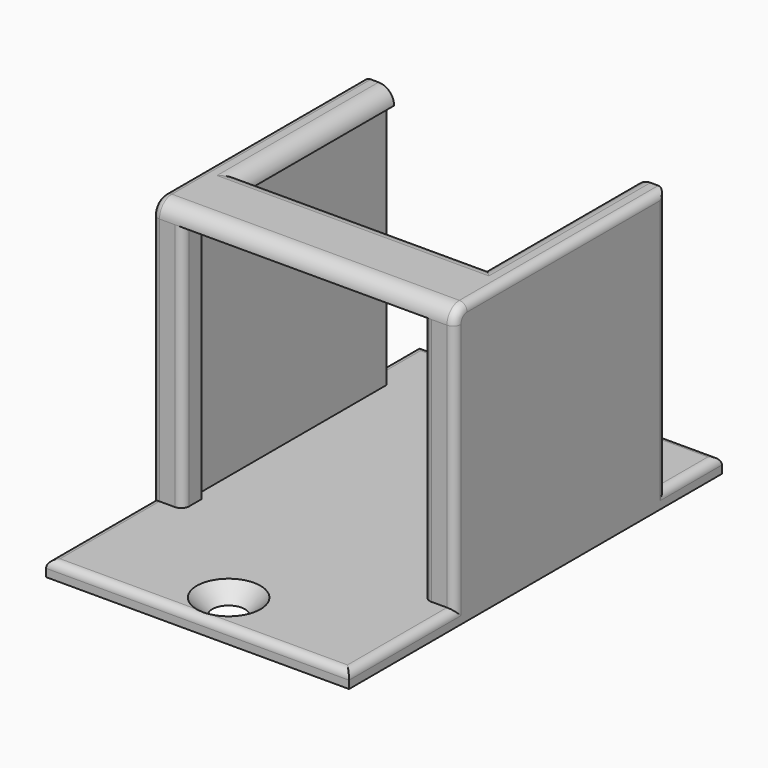
from build123d import *

# Parameters (mm, degrees)
F0_W          = 3
F0_H          = 9
F0_H_2        = 7
F0_H_3        = 3
F0_R          = 2.1
F0_W_2        = 1
F1_DEPTH      = 2
F2_DEPTH      = 34
F3_W          = 4
F3_H          = 2
F4_DEPTH      = 34
F5_SIZE       = 1.99999
F7_W          = 1
F7_H          = 1
F8_DEPTH      = 1
F3_W_2        = 31
F9_DEPTH      = 10
F10_R         = 1.99999
F11_T1_DEPTH  = 32
F11_T3_DEPTH  = 34.50001
F11_T5_DEPTH  = 32.00001
F11_T7_DEPTH  = 19.5
F11_T9_DEPTH  = 11.5
F11_T11_DEPTH = 44
F11_T13_DEPTH = 36.5
F11_T16_ANGLE = 90
F11_T18_ANGLE = 90
F11_T23_DEPTH = 34.50001
F11_T27_DEPTH = 22
F11_T34_DEPTH = 14
F11_T38_DEPTH = 39
F11_T45_DEPTH = 22
F11_T49_DEPTH = 34.50001


# Not quite as in the source:
# - a fillet or chamfer that OpenCascade refuses, or shapes differently, is made with other operations: its cross-section is extruded or revolved along the edge and cut away or added
# - a fillet or chamfer is up to 0.001 mm smaller than in the source, because OpenCascade refuses the exact size
# - a feature of the source that left no trace in its solid (it failed there, or was rolled back) is left out
# - a feature names something its author has since deleted; it is built from what else it names


with BuildPart() as f1:
    # F0 (on Top) → F1 (new body)
    with BuildSketch(Plane.XY):
        with Locations((18, 20.5)):
            Rectangle(F0_W, F0_H)
        with Locations((-18, 20.5)):
            Rectangle(F0_W, F0_H)
        with Locations((18, -21.5)):
            Rectangle(F0_W, F0_H_2)
        with Locations((-18, -21.5)):
            Rectangle(F0_W, F0_H_2)
        with Locations((18, -16.5)):
            Rectangle(F0_W, F0_H_3)
        with Locations((-18, -16.5)):
            Rectangle(F0_W, F0_H_3)
        Polygon((19.5, -35), (19.5, -25), (16.5, -25), (-16.5, -25), (-19.5, -25), (-19.5, -35), align=None)
        with Locations((0, -30)):
            Circle(F0_R, mode=Mode.SUBTRACT)
        Polygon((19.5, -15), (19.5, 16), (16.5, 16), (16.5, 15), (16.5, -15), align=None)
        Polygon((-16.5, 15), (-16.5, 16), (-19.5, 16), (-19.5, 15), (-19.5, -15), (-16.5, -15), align=None)
        Polygon((16.5, 16), (16.5, 25), (-16.5, 25), (-16.5, 16), (-16.5, 15), (16.5, 15), align=None)
        with Locations((0, 20)):
            Circle(F0_R, mode=Mode.SUBTRACT)
        Polygon((16.5, -15), (16.5, 15), (-16.5, 15), (-16.5, -15), (-15.5, -15), (15.5, -15), align=None)
        with Locations((-16, -16.5)):
            Rectangle(F0_W_2, F0_H_3)
        with Locations((16, -16.5)):
            Rectangle(F0_W_2, F0_H_3)
        Polygon((16.5, -25), (16.5, -18), (15.5, -18), (15.5, -15), (-15.5, -15), (-15.5, -18), (-16.5, -18), (-16.5, -25), align=None)
        with Locations((0, -20)):
            Circle(F0_R, mode=Mode.SUBTRACT)
        with Locations((0, -20)):
            Circle(F0_R)
    extrude(amount=-F1_DEPTH)

    # F0 (on Top) → F2 (join)
    with BuildSketch(Plane.XY):
        Polygon((-16.5, 15), (-16.5, 16), (-19.5, 16), (-19.5, 15), (-19.5, -15), (-16.5, -15), align=None)
        with Locations((-18, -16.5)):
            Rectangle(F0_W, F0_H_3)
        with Locations((18, -16.5)):
            Rectangle(F0_W, F0_H_3)
        with Locations((16, -16.5)):
            Rectangle(F0_W_2, F0_H_3)
        with Locations((-16, -16.5)):
            Rectangle(F0_W_2, F0_H_3)
        Polygon((19.5, -15), (19.5, 16), (16.5, 16), (16.5, 15), (16.5, -15), align=None)
    extrude(amount=F2_DEPTH)

    # F3 (on face) → F4 (join)
    with BuildSketch(Plane.XZ.offset(18)):
        with Locations((-17.5, 33)):
            Rectangle(F3_W, F3_H)
        with Locations((17.5, 33)):
            Rectangle(F3_W, F3_H)
    extrude(amount=-F4_DEPTH)

    # F5 (size 2 in the source; OpenCascade refuses exactly that, so slightly less here)
    f5_edges = [f1.edges().sort_by_distance(p)[0] for p in [
        (-2.1, -30, 0),
        (-2.1, 20, 0),
    ]]
    chamfer(f5_edges, length=F5_SIZE)

    # F7 (on face) → F8 (join)
    with BuildSketch(Plane(origin=(0, 16, 0), x_dir=(-1, 0, 0), z_dir=(0, 1, 0))):
        with Locations((-16, 31.5)):
            Rectangle(F7_W, F7_H)
        Polygon((15.9987417102, 33.0025165796), (15.5, 34), (15.5050715785, 33.0000128605), align=None)
    extrude(amount=-F8_DEPTH)

    # F3 (on face) → F9 (join)
    with BuildSketch(Plane.XZ.offset(18)):
        with Locations((0, 33)):
            Rectangle(F3_W_2, F3_H)
    extrude(amount=-F9_DEPTH)

    # F10 (radius 2 in the source; OpenCascade refuses exactly that, so slightly less here)
    f10_edges = [f1.edges().sort_by_distance(p)[0] for p in [
        (0, -18, 34),
        (-15.5, 4, 34),
        (0, -8, 34),
        (15.5, 4, 34),
    ]]
    fillet(f10_edges, radius=F10_R)

    # F11: fillet of radius 1 on 15 edges, made by hand

    # F11_s2 → F11_t1 (cut)
    with BuildSketch(Plane.XY):
        with BuildLine():
            ThreePointArc((-16.5, -18), (-15.7928932188, -17.7071067812), (-15.5, -17))
            Line((-15.5, -17), (-15.5, -18))
            Line((-15.5, -18), (-16.5, -18))
        make_face()
        with BuildLine():
            ThreePointArc((15.5, -17), (15.7928932188, -17.7071067812), (16.5, -18))
            Line((16.5, -18), (15.5, -18))
            Line((15.5, -18), (15.5, -17))
        make_face()
    extrude(amount=F11_T1_DEPTH, mode=Mode.SUBTRACT)

    # F11_s4 → F11_t3 (cut)
    with BuildSketch(Plane.XZ.offset(-18.5)):
        with BuildLine():
            ThreePointArc((-18.5, 34), (-19.2071067812, 33.7071067812), (-19.5, 33))
            Line((-19.5, 33), (-19.5, 34))
            Line((-19.5, 34), (-18.5, 34))
        make_face()
        with BuildLine():
            ThreePointArc((18.5, 34), (19.2071067812, 33.7071067812), (19.5, 33))
            Line((19.5, 33), (19.5, 34))
            Line((19.5, 34), (18.5, 34))
        make_face()
    extrude(amount=F11_T3_DEPTH, mode=Mode.SUBTRACT)

    # F11_s6 → F11_t5 (cut)
    with BuildSketch(Plane.XY):
        with BuildLine():
            ThreePointArc((-19.5, -17), (-19.2071067812, -17.7071067812), (-18.5, -18))
            Line((-18.5, -18), (-19.5, -18))
            Line((-19.5, -18), (-19.5, -17))
        make_face()
        with BuildLine():
            ThreePointArc((18.5, -18), (19.2071067812, -17.7071067812), (19.5, -17))
            Line((19.5, -17), (19.5, -18))
            Line((19.5, -18), (18.5, -18))
        make_face()
    extrude(amount=F11_T5_DEPTH, mode=Mode.SUBTRACT)

    # F11_s8 → F11_t7 (cut)
    with BuildSketch(Plane.XZ.offset(18)):
        with BuildLine():
            ThreePointArc((-19.5, -1), (-19.2071067812, -0.2928932188), (-18.5, 0))
            Line((-18.5, 0), (-19.5, 0))
            Line((-19.5, 0), (-19.5, -1))
        make_face()
        with BuildLine():
            ThreePointArc((18.5, 0), (19.2071067812, -0.2928932188), (19.5, -1))
            Line((19.5, -1), (19.5, 0))
            Line((19.5, 0), (18.5, 0))
        make_face()
    extrude(amount=F11_T7_DEPTH, mode=Mode.SUBTRACT)

    # F11_s10 → F11_t9 (cut)
    with BuildSketch(Plane.XZ.offset(-27.5)):
        with BuildLine():
            ThreePointArc((-19.5, -1), (-19.2071067812, -0.2928932188), (-18.5, 0))
            Line((-18.5, 0), (-19.5, 0))
            Line((-19.5, 0), (-19.5, -1))
        make_face()
        with BuildLine():
            ThreePointArc((18.5, 0), (19.2071067812, -0.2928932188), (19.5, -1))
            Line((19.5, -1), (19.5, 0))
            Line((19.5, 0), (18.5, 0))
        make_face()
    extrude(amount=F11_T9_DEPTH, mode=Mode.SUBTRACT)

    # F11_s12 → F11_t11 (cut)
    with BuildSketch(Plane.YZ.offset(-22)):
        with BuildLine():
            ThreePointArc((-34, 0), (-34.7071067812, -0.2928932188), (-35, -1))
            Line((-35, -1), (-35, 0))
            Line((-35, 0), (-34, 0))
        make_face()
        with BuildLine():
            ThreePointArc((24, 0), (24.7071067812, -0.2928932188), (25, -1))
            Line((25, -1), (25, 0))
            Line((25, 0), (24, 0))
        make_face()
    extrude(amount=F11_T11_DEPTH, mode=Mode.SUBTRACT)

    # F11_s14 → F11_t13 (cut)
    with BuildSketch(Plane.XY):
        with BuildLine():
            ThreePointArc((19.5, 15), (19.2071067812, 15.7071067812), (18.5, 16))
            Line((18.5, 16), (19.5, 16))
            Line((19.5, 16), (19.5, 15))
        make_face()
    extrude(amount=F11_T13_DEPTH, mode=Mode.SUBTRACT)

    # F11_s15 → F11_t16 (revolve, cut)
    with BuildSketch(Plane.XZ.offset(16.00001)):
        with BuildLine():
            ThreePointArc((-19.5, 33), (-19.2071067812, 33.7071067812), (-18.5, 34))
            Line((-18.5, 34), (-19.5, 34))
            Line((-19.5, 34), (-19.5, 33))
        make_face()
    revolve(axis=Axis((-19.5, -16.00001, 32.00001), (1, 0, 0)), revolution_arc=F11_T16_ANGLE, mode=Mode.SUBTRACT)

    # F11_s17 → F11_t18 (revolve, cut)
    with BuildSketch(Plane.XZ.offset(16.00001)):
        with BuildLine():
            ThreePointArc((18.5, 34), (19.2071067812, 33.7071067812), (19.5, 33))
            Line((19.5, 33), (19.5, 34))
            Line((19.5, 34), (18.5, 34))
        make_face()
    revolve(axis=Axis((19.5, -16.00001, 32.00001), (1, 0, 0)), revolution_arc=F11_T18_ANGLE, mode=Mode.SUBTRACT)


with BuildPart() as f11_tool21:
    # F11_s22 → F11_t23 (new body)
    with BuildSketch(Plane.XY.offset(-2.5)):
        with BuildLine():
            ThreePointArc((-19.5, -17), (-19.2071067812, -17.7071067812), (-18.5, -18))
            Line((-18.5, -18), (-19.5, -18))
            Line((-19.5, -18), (-19.5, -17))
        make_face()
    extrude(amount=F11_T23_DEPTH)

    split(bisect_by=Plane.XY, keep=Keep.BOTTOM)


with BuildPart() as f11_tool25:
    # F11_s26 → F11_t27 (new body)
    with BuildSketch(Plane.XZ.offset(15.5)):
        with BuildLine():
            ThreePointArc((-19.5, -1), (-19.2071067812, -0.2928932188), (-18.5, 0))
            Line((-18.5, 0), (-19.5, 0))
            Line((-19.5, 0), (-19.5, -1))
        make_face()
    extrude(amount=F11_T27_DEPTH)

    split(bisect_by=Plane.XZ.offset(18), keep=Keep.BOTTOM)


with BuildPart() as f11_tool21_1:
    add(f11_tool21.part)

    # F11_t29: intersect F11_tool25
    add(f11_tool25.part, mode=Mode.INTERSECT)


with BuildPart() as f1_1:
    add(f1.part)

    # F11_t19: cut F11_tool21
    add(f11_tool21_1.part, mode=Mode.SUBTRACT)


with BuildPart() as f11_tool32:
    # F11_s33 → F11_t34 (new body)
    with BuildSketch(Plane.XZ.offset(-13.5)):
        with BuildLine():
            ThreePointArc((18.5, 0), (19.2071067812, -0.2928932188), (19.5, -1))
            Line((19.5, -1), (19.5, 0))
            Line((19.5, 0), (18.5, 0))
        make_face()
    extrude(amount=-F11_T34_DEPTH)

    split(bisect_by=Plane.XZ.offset(-16), keep=Keep.TOP)


with BuildPart() as f11_tool36:
    # F11_s37 → F11_t38 (new body)
    with BuildSketch(Plane.XY.offset(-2.5)):
        with BuildLine():
            ThreePointArc((19.5, 15), (19.2071067812, 15.7071067812), (18.5, 16))
            Line((18.5, 16), (19.5, 16))
            Line((19.5, 16), (19.5, 15))
        make_face()
    extrude(amount=F11_T38_DEPTH)

    split(bisect_by=Plane.XY, keep=Keep.BOTTOM)


with BuildPart() as f11_tool32_1:
    add(f11_tool32.part)

    # F11_t40: intersect F11_tool36
    add(f11_tool36.part, mode=Mode.INTERSECT)


with BuildPart() as f1_2:
    add(f1_1.part)

    # F11_t30: cut F11_tool32
    add(f11_tool32_1.part, mode=Mode.SUBTRACT)


with BuildPart() as f11_tool43:
    # F11_s44 → F11_t45 (new body)
    with BuildSketch(Plane.XZ.offset(37.5)):
        with BuildLine():
            ThreePointArc((18.5, 0), (19.2071067812, -0.2928932188), (19.5, -1))
            Line((19.5, -1), (19.5, 0))
            Line((19.5, 0), (18.5, 0))
        make_face()
    extrude(amount=-F11_T45_DEPTH)

    split(bisect_by=Plane.XZ.offset(18), keep=Keep.BOTTOM)


with BuildPart() as f11_tool47:
    # F11_s48 → F11_t49 (new body)
    with BuildSketch(Plane.XY.offset(32.00001)):
        with BuildLine():
            ThreePointArc((18.5, -18), (19.2071067812, -17.7071067812), (19.5, -17))
            Line((19.5, -17), (19.5, -18))
            Line((19.5, -18), (18.5, -18))
        make_face()
    extrude(amount=-F11_T49_DEPTH)

    split(bisect_by=Plane.XY, keep=Keep.BOTTOM)


with BuildPart() as f11_tool43_1:
    add(f11_tool43.part)

    # F11_t51: intersect F11_tool47
    add(f11_tool47.part, mode=Mode.INTERSECT)


with BuildPart() as f1_3:
    add(f1_2.part)

    # F11_t41: cut F11_tool43
    add(f11_tool43_1.part, mode=Mode.SUBTRACT)


solid = f1_3.part
